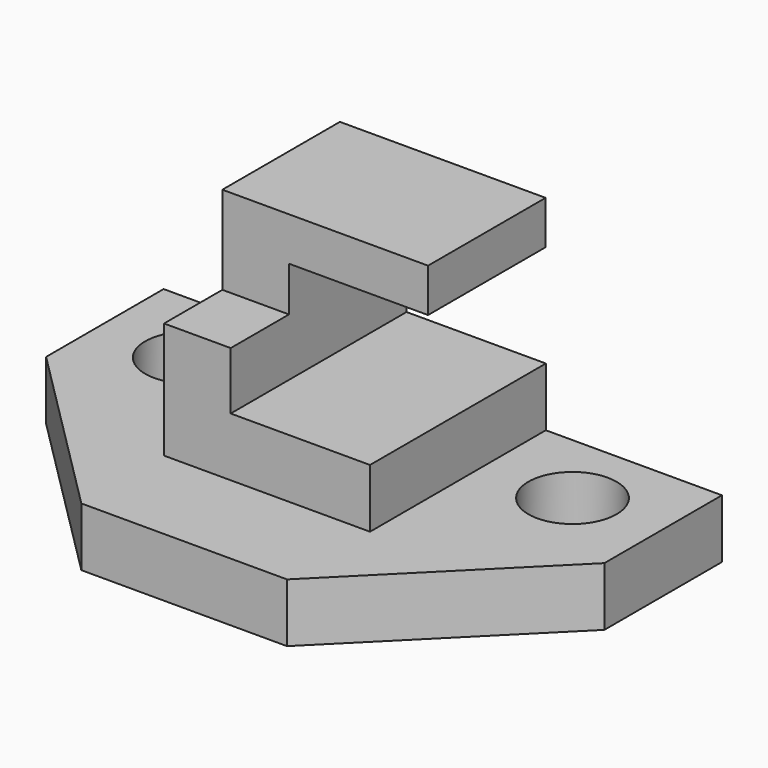
from build123d import *

# Parameters (mm, degrees)
F0_R     = 9.525
F1_DEPTH = 12.7
F3_DEPTH = 47.498
F4_DEPTH = 31.75


# Not quite as in the source:
# - a feature names something its author has since deleted; it is built from what else it names


with BuildPart() as f1:
    # F0 (on Top) → F1 (new body)
    with BuildSketch(Plane.XY):
        Polygon((68.1566672574, 0), (-52.4933327426, 0), (-52.4933327426, -31.75), (-14.3933327426, -69.85), (30.0566672574, -69.85), (68.1566672574, -31.75), align=None)
        with Locations((-33.4641109884, -16.8546829373)):
            Circle(F0_R, mode=Mode.SUBTRACT)
        with Locations((49.0858890116, -16.5274422616)):
            Circle(F0_R, mode=Mode.SUBTRACT)
    extrude(amount=F1_DEPTH)

    # F2 (on Front) → F3 (join)
    with BuildSketch(Plane.XZ):
        Polygon((-14.398525469, 37.846), (-14.3439900845, 0), (30.1060099155, 0), (30.1060099155, 25.4), (0, 25.4), (0, 37.846), align=None)
    extrude(amount=F3_DEPTH)

    # F2 (on Front) → F4 (join)
    with BuildSketch(Plane.XZ):
        Polygon((-14.398525469, 56.896), (-14.398525469, 37.846), (0, 37.846), (0, 47.498), (30.051474531, 47.498), (30.051474531, 56.896), align=None)
    extrude(amount=F4_DEPTH)


solid = f1.part
